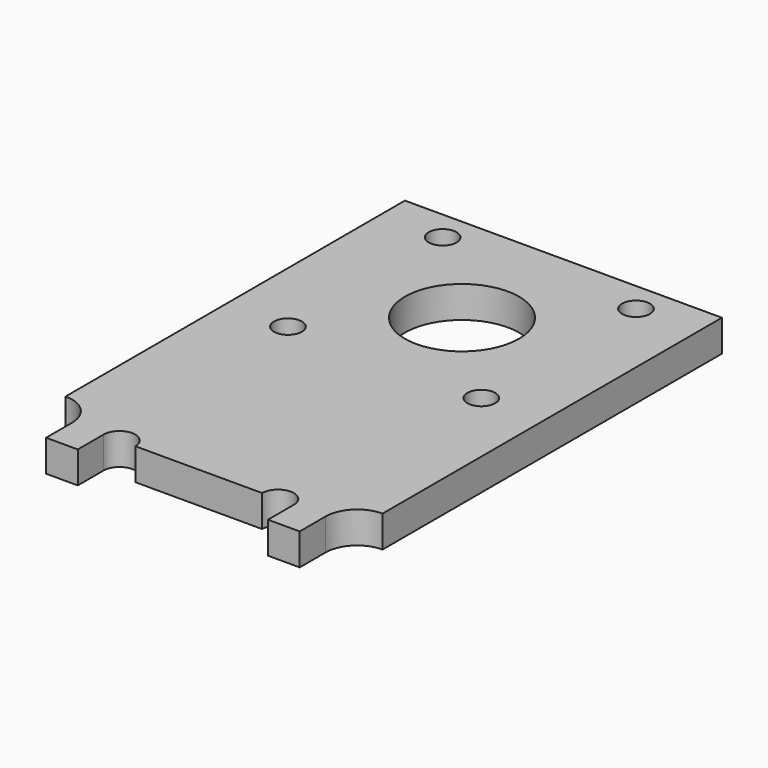
from build123d import *

# Parameters (mm, degrees)
F1_R     = 2.2
F1_R_2   = 9
F2_DEPTH = 5


# Not quite as in the source:
# - a feature names something its author has since deleted; it is built from what else it names


with BuildPart() as f2:
    # F1 (on Top) → F2 (new body)
    with BuildSketch(Plane.XY):
        with BuildLine():
            Line((25, 20), (20, 20))
            Line((20, 20), (-20, 20))
            Line((-20, 20), (-25, 20))
            Line((-25, 20), (-25, -46.9))
            ThreePointArc((-25, -46.9), (-21.4644660941, -48.3644660941), (-20, -51.9))
            Line((-20, -51.9), (-20, -57))
            Line((-20, -57), (-15, -57))
            Line((-15, -57), (-15, -51.9))
            ThreePointArc((-15, -51.9), (-12.5, -49.4), (-10, -51.9))
            Line((-10, -51.9), (0, -51.9))
            Line((0, -51.9), (10, -51.9))
            ThreePointArc((10, -51.9), (12.5, -49.4), (15, -51.9))
            Line((15, -51.9), (15, -57))
            Line((15, -57), (20, -57))
            Line((20, -57), (20, -51.9))
            ThreePointArc((20, -51.9), (21.4644660941, -48.3644660941), (25, -46.9))
            Line((25, -46.9), (25, 20))
        make_face()
        with Locations((-15.25, -15.25)):
            Circle(F1_R, mode=Mode.SUBTRACT)
        with Locations((-15.25, 15.25)):
            Circle(F1_R, mode=Mode.SUBTRACT)
        Circle(F1_R_2, mode=Mode.SUBTRACT)
        with Locations((15.25, -15.25)):
            Circle(F1_R, mode=Mode.SUBTRACT)
        with Locations((15.25, 15.25)):
            Circle(F1_R, mode=Mode.SUBTRACT)
    extrude(amount=F2_DEPTH)


solid = f2.part
